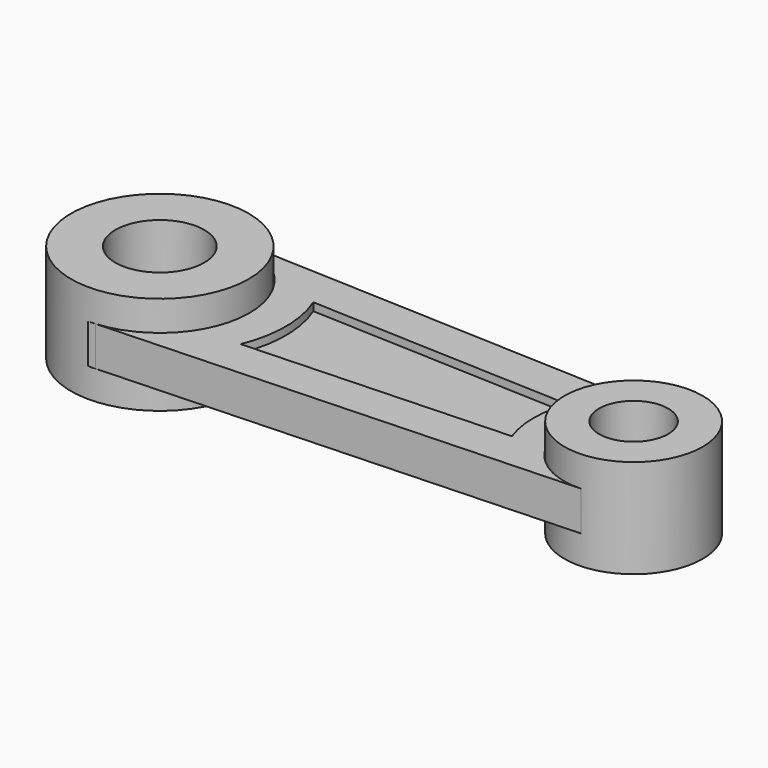
from build123d import *

# Parameters (mm, degrees)
F0_R     = 56.25
F0_R_2   = 28.15
F1_DEPTH = 31.25
F0_R_3   = 43.75
F0_R_4   = 21.9
F3_DEPTH = 12.5
F5_DEPTH = 5


# Not quite as in the source:
# - a pattern or mirror of a feature is missing from the dataset's text; its kind, count and spacing are read off the source's solid


with BuildPart() as f1:
    # F0 (on Top) → F1 (new body, symmetric)
    with BuildSketch(Plane.XY):
        Circle(F0_R)
        Circle(F0_R_2, mode=Mode.SUBTRACT)
    extrude(amount=F1_DEPTH, both=True)


with BuildPart() as f1b:
    # F0 (on Top) → F1, piece 2 (new body, symmetric)
    with BuildSketch(Plane.XY):
        with Locations((300, 0)):
            Circle(F0_R_3)
        with Locations((300, 0)):
            Circle(F0_R_4, mode=Mode.SUBTRACT)
    extrude(amount=F1_DEPTH, both=True)


with BuildPart() as f3:
    # F2 (on Top) → F3 (new body, symmetric)
    with BuildSketch(Plane.XY):
        with BuildLine():
            Line((4.6259014272, -56.5867262298), (0, -56.7754925071))
            ThreePointArc((0, -56.7754925071), (2.3148756296, -56.7282813087), (4.6259014272, -56.5867262298))
        make_face()
    extrude(amount=F3_DEPTH, both=True)


with BuildPart() as f3b:
    # F2 (on Top) → F3, piece 2 (new body, symmetric)
    with BuildSketch(Plane.XY):
        with BuildLine():
            Line((0, 56.7754925071), (4.6259014272, 56.5867262298))
            ThreePointArc((4.6259014272, 56.5867262298), (2.3148756296, 56.7282813087), (0, 56.7754925071))
        make_face()
    extrude(amount=F3_DEPTH, both=True)


with BuildPart() as f3c:
    # F2 (on Top) → F3, piece 3 (new body, symmetric)
    with BuildSketch(Plane.XY):
        with BuildLine():
            ThreePointArc((4.6259014272, 56.5867262298), (56.7754925071, 0), (4.6259014272, -56.5867262298))
            Line((4.6259014272, -56.5867262298), (302.1896357559, -44.4442283265))
            ThreePointArc((302.1896357559, -44.4442283265), (255.8948115028, 0), (302.1896357559, 44.4442283265))
            Line((302.1896357559, 44.4442283265), (4.6259014272, 56.5867262298))
        make_face()
    extrude(amount=F3_DEPTH, both=True)

    # F4 (on face) → F5 (cut)
    with BuildSketch(Plane.XY.offset(12.5)):
        with BuildLine():
            ThreePointArc((74.1885877339, 28.7273191849), (79.8071242601, 0), (74.1885877339, -28.7273191849))
            Line((74.1885877339, -28.7273191849), (240.5203489402, -21.9399226419))
            ThreePointArc((240.5203489402, -21.9399226419), (236.6260278225, 0), (240.5203489402, 21.9399226419))
            Line((240.5203489402, 21.9399226419), (74.1885877339, 28.7273191849))
        make_face()
    f5 = extrude(amount=-F5_DEPTH, mode=Mode.SUBTRACT)

    # F5_copies: F5 across plane
    add(f5.mirror(Plane(origin=(0, 0, 0), x_dir=(-1, 0, 0), z_dir=(0, 0, -1))), mode=Mode.SUBTRACT)


solid = Compound([f1.part, f1b.part, f3.part, f3b.part, f3c.part])
